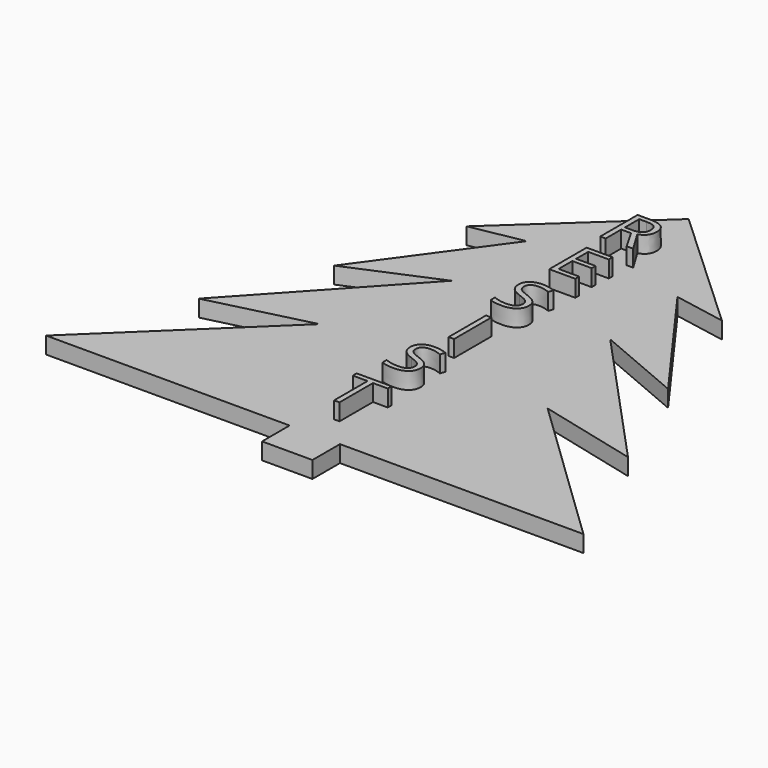
from build123d import *

# Parameters (mm, degrees)
F1_DEPTH       = 1
F2_TEXT_SIZE   = 3.911422876
F2_TEXT_SIZE_2 = 3.9114166667
F3_DEPTH       = 1


# Not quite as in the source:
# - Text() gives the source's letters only with a copy of the font that has no kerning and outlines rounded to 1/6400 em; it was checked with that copy


with BuildPart() as f1:
    # F0 (on Top) → F1 (new body)
    with BuildSketch(Plane.XY):
        Polygon((7.6306981817, 22.9510784138), (0, 30), (-7.6306981817, 22.9510784138), (-4.5106832273, 23.5288567838), (-9.9808432404, 15.9865699188), (-4.7417960448, 18.2132761858), (-12.8307231057, 9.4310126317), (-6.8218055246, 10.9332412922), (-16.0662937341, 2.0573371113), (-13.7155810683, 2.0573371113), (-1.5062228447, 2.0573371113), (-1.5062228447, 0), (0, 0), (1.5062228447, 0), (1.5062228447, 2.0573371113), (13.7155810683, 2.0573371113), (16.0662937341, 2.0573371113), (6.8218055246, 10.9332412922), (12.8307231057, 9.4310126317), (4.7417960448, 18.2132761858), (9.9808432404, 15.9865699188), (4.5106832273, 23.5288567838), align=None)
    extrude(amount=F1_DEPTH)

    # F2 (on face) → F3 (join)
    with BuildSketch(Plane.XY.offset(1)):
        with Locations((-1.3023815857, 24.5438739657)):
            Text('R', F2_TEXT_SIZE, font='Open Sans', text_align=(TextAlign.LEFT, TextAlign.BOTTOM))
        with Locations((-1.0970301432, 20.4759992663)):
            Text('E', F2_TEXT_SIZE_2, font='Open Sans', text_align=(TextAlign.LEFT, TextAlign.BOTTOM))
        with Locations((-0.4809820182, 12.18378)):
            Text('I', F2_TEXT_SIZE_2, font='Open Sans', text_align=(TextAlign.LEFT, TextAlign.BOTTOM))
        with Locations((-1.1065031055, 16.2516597662)):
            Text('S', F2_TEXT_SIZE_2, font='Open Sans', text_align=(TextAlign.LEFT, TextAlign.BOTTOM))
        with Locations((-1.1905374479, 3.8394078616)):
            Text('T', F2_TEXT_SIZE_2, font='Open Sans', text_align=(TextAlign.LEFT, TextAlign.BOTTOM))
        with Locations((-1.1065031055, 8.1615299454)):
            Text('S', F2_TEXT_SIZE_2, font='Open Sans', text_align=(TextAlign.LEFT, TextAlign.BOTTOM))
    extrude(amount=F3_DEPTH)


solid = f1.part
